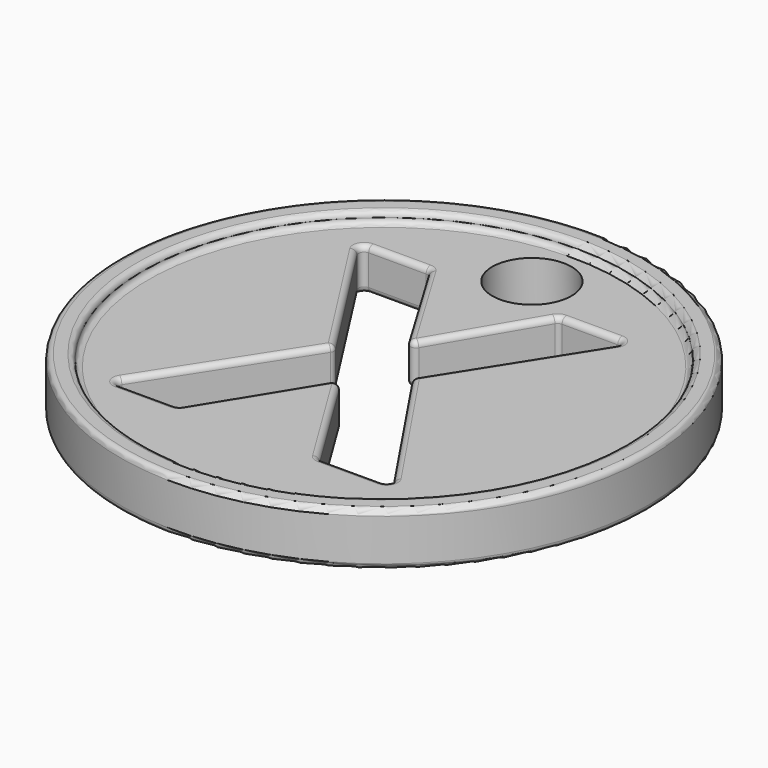
from build123d import *

# Parameters (mm, degrees)
F2_TEXT_SIZE = 18.7783110325
F3_DEPTH     = 25
F4_R         = 0.24999
F6_D         = 3.5


# Not quite as in the source:
# - a fillet or chamfer is up to 0.001 mm smaller than in the source, because OpenCascade refuses the exact size
# - Text() gives the source's letters only with a copy of the font that has no kerning and outlines rounded to 1/6400 em; it was checked with that copy


with BuildPart() as f1:
    # F0 (on Front) → F1 (revolve)
    with BuildSketch(Plane.XZ):
        Polygon((0, 0.675), (0, -1.175), (11.665, -1.175), (11.665, 1.175), (10.665, 1.175), (10.665, 0.675), align=None)
    revolve(axis=Axis((0, 0, 0.4655460789), (0, 0, -1)))

    # F2 (on face) → F3 (cut)
    with BuildSketch(Plane.XY.offset(0.675)):
        with Locations((-6.7693308235, -6.7206211292)):
            Text('X', F2_TEXT_SIZE, font='Open Sans', font_style=FontStyle.BOLD, text_align=(TextAlign.LEFT, TextAlign.BOTTOM))
    extrude(amount=-F3_DEPTH, mode=Mode.SUBTRACT)

    # F4 (radius 0.25 in the source; OpenCascade refuses exactly that, so slightly less here)
    f4_edges = [f1.edges().sort_by_distance(p)[0] for p in [
        (-11.665, 0, 1.175),
        (-4.40297, 3.438739, 0.675),
        (-11.665, 0, -1.175),
        (-10.665, 0, 1.175),
        (-10.665, 0, 0.675),
        (0.951783, -4.185549, 0.675),
        (-1.904575, 4.273493, -1.175),
        (-1.904575, 4.273493, 0.675),
        (3.491256, -3.341992, -1.175),
        (3.903498, 6.685332, 0.675),
        (3.491256, -3.341992, 0.675),
        (-2.165711, -4.185549, 0.675),
        (-5.246527, -6.720621, 0.675),
        (5.756389, -6.720621, -0.25),
        (2.511263, -6.720621, -0.25),
        (-0.607698, -1.650477, -0.25),
        (-3.723724, -6.720621, -0.25),
        (-6.769331, -6.720621, -0.25),
        (-6.484722, 6.685332, -0.25),
        (-3.348157, 6.685332, -0.25),
        (-0.460992, 1.861654, -0.25),
        (2.373359, 6.685332, -0.25),
        (5.433637, 6.685332, -0.25),
        (1.226122, 0.036637, -0.25),
        (4.133826, -6.720621, 0.675),
        (-4.40297, 3.438739, -1.175),
        (-4.91644, 6.685332, -1.175),
        (-4.545275, -3.264238, 0.675),
        (0.956184, 4.273493, -1.175),
        (3.903498, 6.685332, -1.175),
        (-4.91644, 6.685332, 0.675),
        (3.32988, 3.360985, -1.175),
        (0.956184, 4.273493, 0.675),
        (3.32988, 3.360985, 0.675),
        (4.133826, -6.720621, -1.175),
        (0.951783, -4.185549, -1.175),
        (-2.165711, -4.185549, -1.175),
        (-5.246527, -6.720621, -1.175),
        (-4.545275, -3.264238, -1.175),
        (-2.321218, 0.192145, -0.25),
    ]]
    fillet(f4_edges, radius=F4_R)

    # F6 (through all)
    with Locations(Plane.XY.offset(0.675)):
        with Locations((0, 8.165)):
            Hole(F6_D / 2)


solid = f1.part
